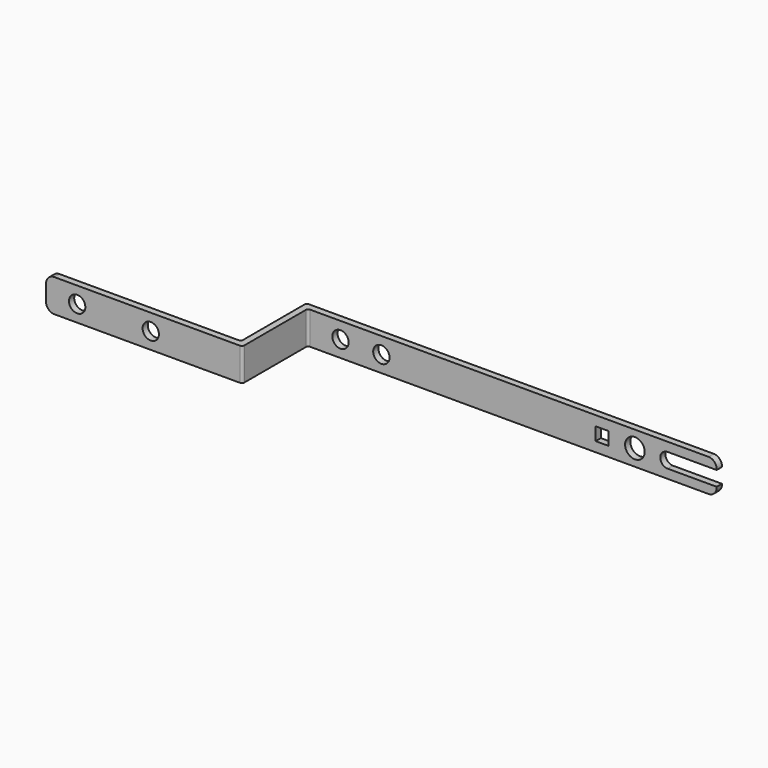
from build123d import *

# Parameters (mm, degrees)
F2_DEPTH = 10
F3_R     = 5
F3_R_2   = 6
F3_W     = 8
F3_H     = 8
F4_DEPTH = 54.001
F5_R     = 5
F6_R     = 1.5


with BuildPart() as f2:
    # F1 (on Top) → F2 (new body, symmetric)
    with BuildSketch(Plane.XY):
        Polygon((0, 0), (0, 50), (250, 50), (250, 54), (-4, 54), (-4, 4), (-120, 4), (-120, 0), align=None)
    extrude(amount=F2_DEPTH, both=True)

    # F3 (on Front) → F4 (cut, through all)
    with BuildSketch(Plane.XZ):
        with Locations((-101, 0)):
            Circle(F3_R)
        with Locations((-56, 0)):
            Circle(F3_R)
        with Locations((20, 0)):
            Circle(F3_R)
        with Locations((45, 0)):
            Circle(F3_R)
        with Locations((200, 0)):
            Circle(F3_R_2)
        with BuildLine():
            ThreePointArc((220, -4.5), (223.1819805153, -3.1819805153), (224.5, 0))
            ThreePointArc((224.5, 0), (223.1819805153, 3.1819805153), (220, 4.5))
            ThreePointArc((220, 4.5), (215.5, 0), (220, -4.5))
        make_face()
        with BuildLine():
            ThreePointArc((220, 4.5), (223.1819805153, 3.1819805153), (224.5, 0))
            ThreePointArc((224.5, 0), (223.1819805153, -3.1819805153), (220, -4.5))
            Line((220, -4.5), (250, -4.5))
            Line((250, -4.5), (250, 4.5))
            Line((250, 4.5), (220, 4.5))
        make_face()
        with Locations((180, 0)):
            Rectangle(F3_W, F3_H)
    extrude(amount=-F4_DEPTH, mode=Mode.SUBTRACT)

    # F5
    f5_edges = [f2.edges().sort_by_distance(p)[0] for p in [
        (-120, 2, 10),
        (-120, 2, -10),
        (250, 52, -10),
        (250, 52, 10),
    ]]
    fillet(f5_edges, radius=F5_R)

    # F6
    f6_edges = [f2.edges().sort_by_distance(p)[0] for p in [
        (-4, 54, 0),
        (0, 50, 0),
        (0, 0, 0),
        (-4, 4, 0),
    ]]
    fillet(f6_edges, radius=F6_R)


solid = f2.part
